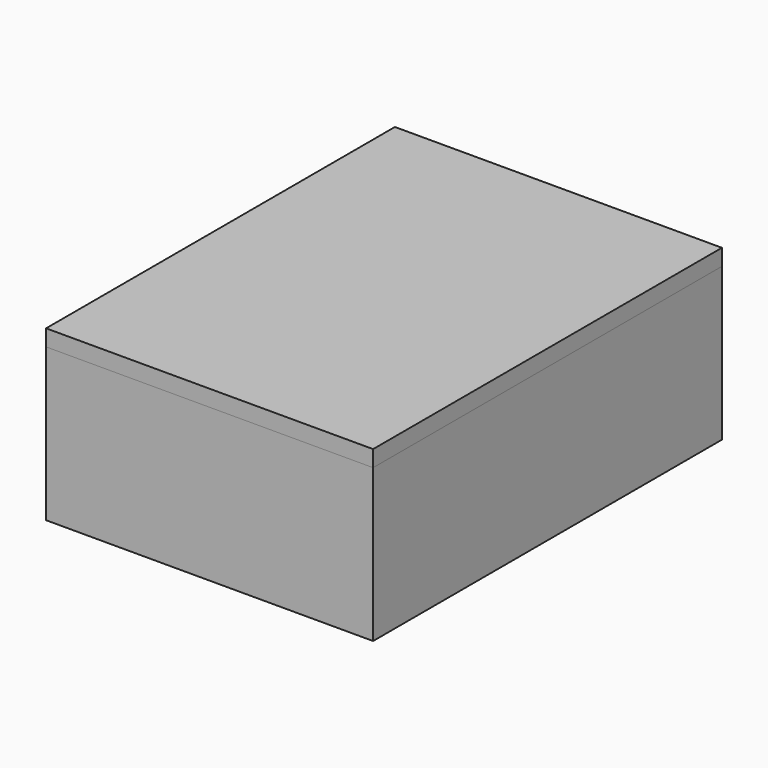
from build123d import *

# Parameters (mm, degrees)
F0_W     = 60
F0_H     = 80
F1_DEPTH = 25
F2_T     = -3
F4_DEPTH = 3
F3_W     = 60
F3_H     = 80
F3_W_2   = 54
F3_H_2   = 74
F6_DEPTH = 3
F5_W     = 53.7855226994
F5_H     = 73.69507429
F7_DEPTH = 4


# Not quite as in the source:
# - the program builds the solid bodies; features that only make, move or delete a surface that nothing else refers to are left out


with BuildPart() as f1:
    # F0 (on Top) → F1 (new body)
    with BuildSketch(Plane.XY):
        Rectangle(F0_W, F0_H)
    extrude(amount=F1_DEPTH)

    # F2
    f2_openings = [f1.faces().sort_by_distance(p)[0] for p in [
        (0, 0, 25),
    ]]
    offset(amount=F2_T, openings=f2_openings)

    # F4 (add): a face of the model
    f4_faces = [f1.faces().sort_by_distance(p)[0] for p in [
        (0, 0, 0),
    ]]
    extrude(f4_faces, amount=F4_DEPTH)


with BuildPart() as f6:
    # F3 (on face) → F6 (new body)
    with BuildSketch(Plane.XY.offset(25)):
        Rectangle(F3_W, F3_H)
        Rectangle(F3_W_2, F3_H_2, mode=Mode.SUBTRACT)
        Rectangle(F3_W_2, F3_H_2)
    extrude(amount=F6_DEPTH)

    # F5 (on face) → F7 (join)
    with BuildSketch(Plane.XY.offset(25)):
        with Locations((-0.1072386503, -0.152462855)):
            Rectangle(F5_W, F5_H)
    extrude(amount=-F7_DEPTH)


solid = Compound([f1.part, f6.part])
